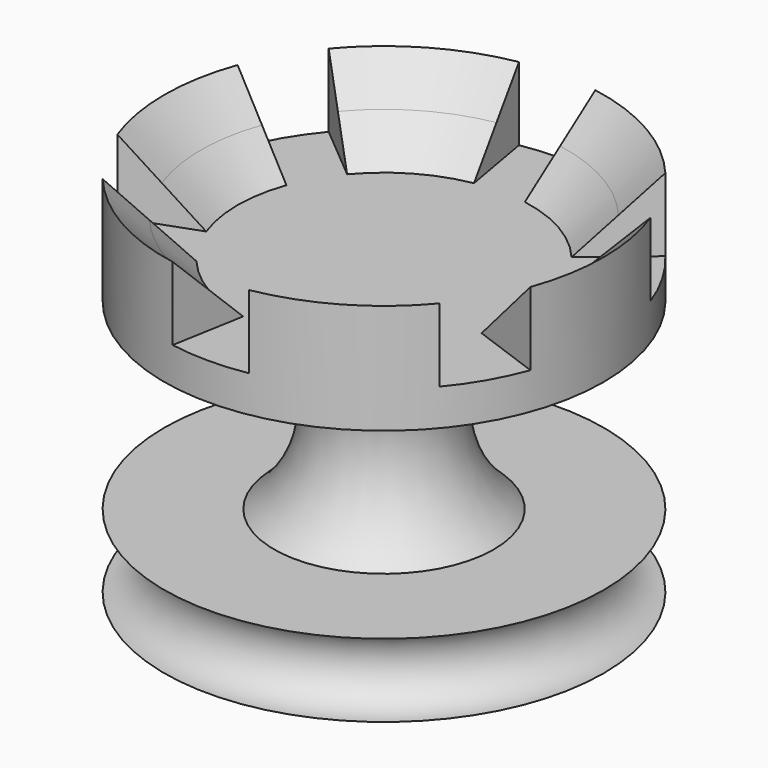
from build123d import *

# Parameters (mm, degrees)
F2_R     = 25
F3_DEPTH = 10
F5_DEPTH = 42.2
F6_SIZE  = 4.99999


# Not quite as in the source:
# - a fillet or chamfer is up to 0.001 mm smaller than in the source, because OpenCascade refuses the exact size


with BuildPart() as f1:
    # F0 (on Front) → F1 (revolve)
    with BuildSketch(Plane.XZ):
        with BuildLine():
            Line((0, 10), (0, 0))
            Line((0, 0), (15, 0))
            Line((15, 0), (30, 0))
            ThreePointArc((30, 0), (25, 5), (30, 10))
            Line((30, 10), (15, 10))
            ThreePointArc((15, 10), (9.1886000762, 22.5), (15, 35))
            Line((15, 35), (30, 35))
            Line((30, 35), (30, 50))
            Line((30, 50), (0, 50))
            Line((0, 50), (0, 35))
            Line((0, 35), (0, 10))
        make_face()
    revolve(axis=Axis((0, 0, 42.5), (0, 0, 1)))

    # F2 (on face) → F3 (cut)
    with BuildSketch(Plane.XY.offset(50)):
        Circle(F2_R)
    extrude(amount=-F3_DEPTH, mode=Mode.SUBTRACT)

    # F4 (on face) → F5 (cut)
    with BuildSketch(Plane.XY.offset(40)):
        with BuildLine():
            ThreePointArc((-4.3412044417, 24.6201938253), (0, 25), (4.3412044417, 24.6201938253))
            Line((4.3412044417, 24.6201938253), (5.20944533, 29.5442325904))
            ThreePointArc((5.20944533, 29.5442325904), (0, 30), (-5.20944533, 29.5442325904))
            Line((-5.20944533, 29.5442325904), (-4.3412044417, 24.6201938253))
        make_face()
        with BuildLine():
            Line((-19.151111078, 16.0696902422), (-22.9813332936, 19.2836282906))
            ThreePointArc((-22.9813332936, 19.2836282906), (-25.9807621135, 15), (-28.1907786236, 10.2606042998))
            Line((-28.1907786236, 10.2606042998), (-23.4923155196, 8.5505035831))
            ThreePointArc((-23.4923155196, 8.5505035831), (-21.6506350946, 12.5), (-19.151111078, 16.0696902422))
        make_face()
        with BuildLine():
            Line((-23.4923155196, -8.5505035831), (-28.1907786236, -10.2606042998))
            ThreePointArc((-28.1907786236, -10.2606042998), (-25.9807621135, -15), (-22.9813332936, -19.2836282906))
            Line((-22.9813332936, -19.2836282906), (-19.151111078, -16.0696902422))
            ThreePointArc((-19.151111078, -16.0696902422), (-21.6506350946, -12.5), (-23.4923155196, -8.5505035831))
        make_face()
        with BuildLine():
            Line((-4.3412044417, -24.6201938253), (-5.20944533, -29.5442325904))
            ThreePointArc((-5.20944533, -29.5442325904), (0, -30), (5.20944533, -29.5442325904))
            Line((5.20944533, -29.5442325904), (4.3412044417, -24.6201938253))
            ThreePointArc((4.3412044417, -24.6201938253), (0, -25), (-4.3412044417, -24.6201938253))
        make_face()
        with BuildLine():
            Line((19.151111078, -16.0696902422), (22.9813332936, -19.2836282906))
            ThreePointArc((22.9813332936, -19.2836282906), (25.9807621135, -15), (28.1907786236, -10.2606042998))
            Line((28.1907786236, -10.2606042998), (23.4923155196, -8.5505035831))
            ThreePointArc((23.4923155196, -8.5505035831), (21.6506350946, -12.5), (19.151111078, -16.0696902422))
        make_face()
        with BuildLine():
            Line((23.4923155196, 8.5505035831), (28.1907786236, 10.2606042998))
            ThreePointArc((28.1907786236, 10.2606042998), (25.9807621135, 15), (22.9813332936, 19.2836282906))
            Line((22.9813332936, 19.2836282906), (19.151111078, 16.0696902422))
            ThreePointArc((19.151111078, 16.0696902422), (21.6506350946, 12.5), (23.4923155196, 8.5505035831))
        make_face()
    extrude(amount=F5_DEPTH, mode=Mode.SUBTRACT)

    # F6 (size 5 in the source; OpenCascade refuses exactly that, so slightly less here)
    f6_edges = [f1.edges().sort_by_distance(p)[0] for p in [
        (25, 0, 40),
        (-12.5, -21.650635, 40),
        (-25, 0, 40),
        (-12.5, 21.650635, 40),
        (12.5, 21.650635, 40),
        (-12.5, 21.650635, 50),
        (12.5, 21.650635, 50),
        (25, 0, 50),
        (12.5, -21.650635, 40),
        (12.5, -21.650635, 50),
        (-12.5, -21.650635, 50),
        (-25, 0, 50),
    ]]
    chamfer(f6_edges, length=F6_SIZE)


solid = f1.part
